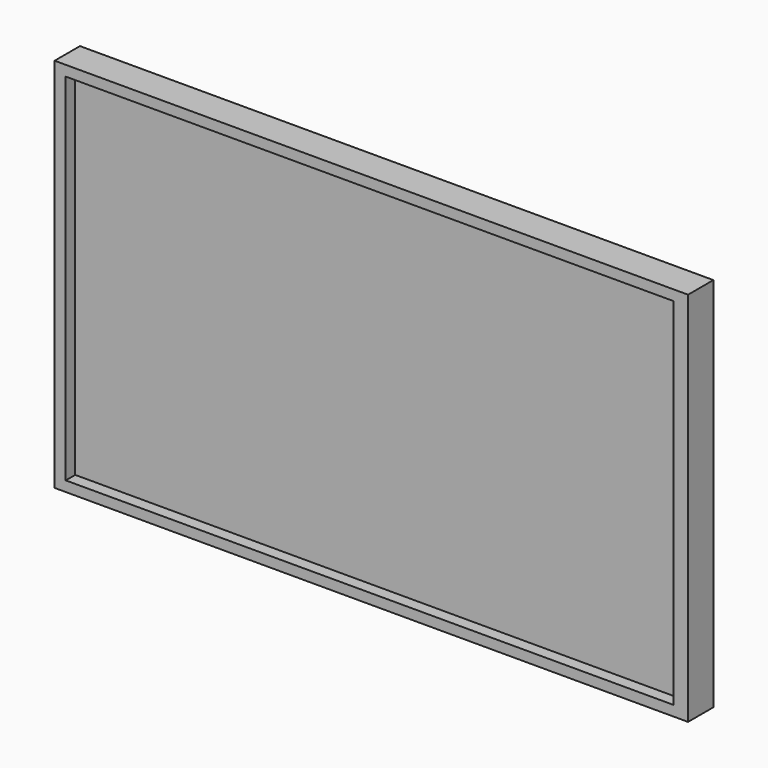
from build123d import *

# Parameters (mm, degrees)
F0_W     = 160
F0_H     = 95
F1_DEPTH = 8
F2_W     = 153.534181416
F2_H     = 89.7976644337
F3_DEPTH = 3
F4_W     = 75.6339989603
F4_H     = 27.7607943863
F5_DEPTH = 16
F6_R     = 5


with BuildPart() as f1:
    # F0 (on Front) → F1 (new body)
    with BuildSketch(Plane.XZ):
        with Locations((4.0975642204, 18.1421419978)):
            Rectangle(F0_W, F0_H)
    extrude(amount=F1_DEPTH)

    # F2 (on face) → F3 (cut)
    with BuildSketch(Plane.XZ.offset(8)):
        with Locations((3.6726556718, 18.1294959038)):
            Rectangle(F2_W, F2_H)
    extrude(amount=-F3_DEPTH, mode=Mode.SUBTRACT)

    # F4 (on face) → F5 (join)
    with BuildSketch(Plane(origin=(0, 0, 0), x_dir=(-1, 0, 0), z_dir=(0, 1, 0))):
        with Locations((-5.2306558937, 21.3871421292)):
            Rectangle(F4_W, F4_H)
    extrude(amount=F5_DEPTH)

    # F6
    f6_edges = [f1.edges().sort_by_distance(p)[0] for p in [
        (-32.586344, 8, 35.267539),
        (43.047655, 8, 35.267539),
        (5.230656, 0, 35.267539),
        (5.230656, 16, 35.267539),
        (43.047655, 8, 7.506745),
        (-32.586344, 8, 7.506745),
        (5.230656, 0, 7.506745),
        (5.230656, 16, 7.506745),
        (-32.586344, 0, 21.387142),
        (43.047655, 0, 21.387142),
    ]]
    fillet(f6_edges, radius=F6_R)


solid = f1.part
